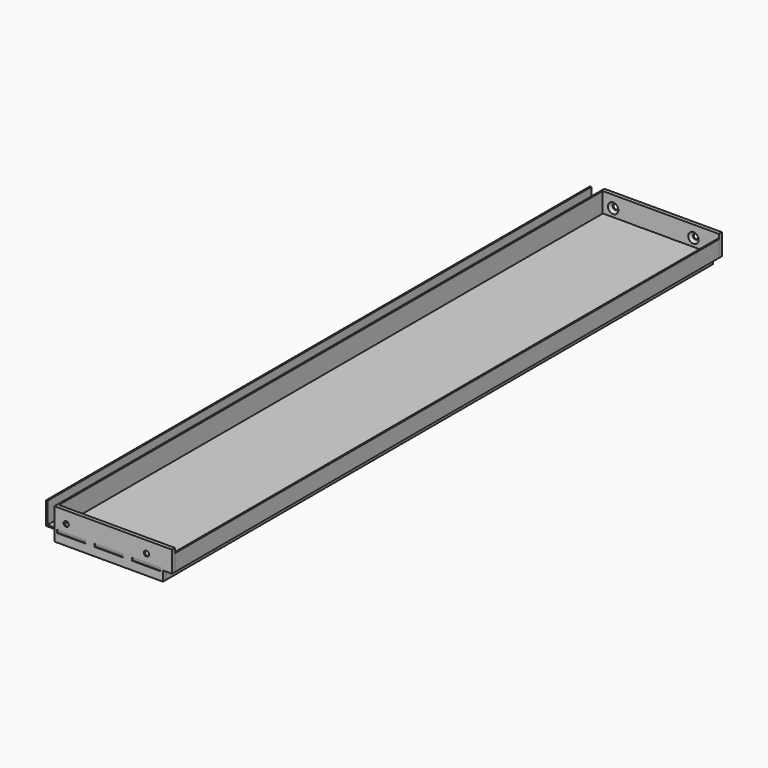
from build123d import *

# Parameters (mm, degrees)
F1_DEPTH        = 1440
F2_DEPTH        = 1440
F3_W            = 60
F3_H            = 7
F4_DEPTH        = 3
F6_W            = 60
F6_H            = 7
F7_DEPTH        = 3
F8_W            = 60.5
F8_H            = 6.5
F9_DEPTH        = 8
F12_D           = 11
F12_CSINK_D     = 22
F12_CSINK_ANGLE = 90
F14_D           = 11
F14_CSINK_D     = 22
F14_CSINK_ANGLE = 90


with BuildPart() as f1:
    # F0 (on Front) → F1 (new body)
    with BuildSketch(Plane.XZ):
        Polygon((3, 48), (0, 48), (0, 0), (251, 0), (251, -18), (254, -18), (254, 3), (24, 3), (3, 3), align=None)
    extrude(amount=-F1_DEPTH)

    # F6 (on face) → F7 (join)
    with BuildSketch(Plane(origin=(0, 0, 0), x_dir=(1, 0, 0), z_dir=(0, 0, -1))):
        with Locations((219, 3.5)):
            Rectangle(F6_W, F6_H)
        with Locations((139.5732760429, 3.5)):
            Rectangle(F6_W, F6_H)
        with Locations((59.5732760429, 3.5)):
            Rectangle(F6_W, F6_H)
        with Locations((219, -1443.5)):
            Rectangle(F6_W, F6_H)
        with Locations((59.5732760429, -1443.5)):
            Rectangle(F6_W, F6_H)
        with Locations((139.5732760429, -1443.5)):
            Rectangle(F6_W, F6_H)
    extrude(amount=-F7_DEPTH)


with BuildPart() as f2:
    # F0 (on Front) → F2 (new body)
    with BuildSketch(Plane.XZ):
        Polygon((24, 48), (24, 3), (254, 3), (273, 3), (273, 6), (273, 38), (270, 38), (270, 6), (27, 6), (27, 48), align=None)
    extrude(amount=-F2_DEPTH)

    # F3 (on face) → F4 (join)
    with BuildSketch(Plane(origin=(0, 0, 3), x_dir=(1, 0, 0), z_dir=(0, 0, -1))):
        with Locations((59.5732760429, 3.5)):
            Rectangle(F3_W, F3_H)
        with Locations((139.5732760429, 3.5)):
            Rectangle(F3_W, F3_H)
        with Locations((219, 3.5)):
            Rectangle(F3_W, F3_H)
        with Locations((219, -1443.5)):
            Rectangle(F3_W, F3_H)
        with Locations((59.5732760429, -1443.5)):
            Rectangle(F3_W, F3_H)
        with Locations((139.5732760429, -1443.5)):
            Rectangle(F3_W, F3_H)
    extrude(amount=-F4_DEPTH)


with BuildPart() as f9:
    # F8 (on face) → F9 (new body)
    with BuildSketch(Plane.XZ):
        Polygon((254, 3), (273, 3), (273, 48), (24, 48), (24, -18), (254, -18), align=None)
        with Locations((59.5732760429, 3)):
            Rectangle(F8_W, F8_H, mode=Mode.SUBTRACT)
        with Locations((139.5732760429, 3)):
            Rectangle(F8_W, F8_H, mode=Mode.SUBTRACT)
        with Locations((219, 3)):
            Rectangle(F8_W, F8_H, mode=Mode.SUBTRACT)
    extrude(amount=F9_DEPTH)


with BuildPart() as f10_1:
    # F10: instance of F9
    add(f9.part.mirror(Plane.XZ.offset(-720)))

    # F14 (through all)
    with Locations(Plane.XZ.offset(-1440)):
        with Locations((49, 23), (219, 23)):
            CounterSinkHole(F14_D / 2, F14_CSINK_D / 2, counter_sink_angle=F14_CSINK_ANGLE)


with BuildPart() as f9_1:
    add(f9.part)

    # F12 (through all)
    with Locations(Plane(origin=(0, 0, 0), x_dir=(-1, 0, 0), z_dir=(0, 1, 0))):
        with Locations((-49, 23), (-219, 23)):
            CounterSinkHole(F12_D / 2, F12_CSINK_D / 2, counter_sink_angle=F12_CSINK_ANGLE)


solid = Compound([f1.part, f2.part, f10_1.part, f9_1.part])
